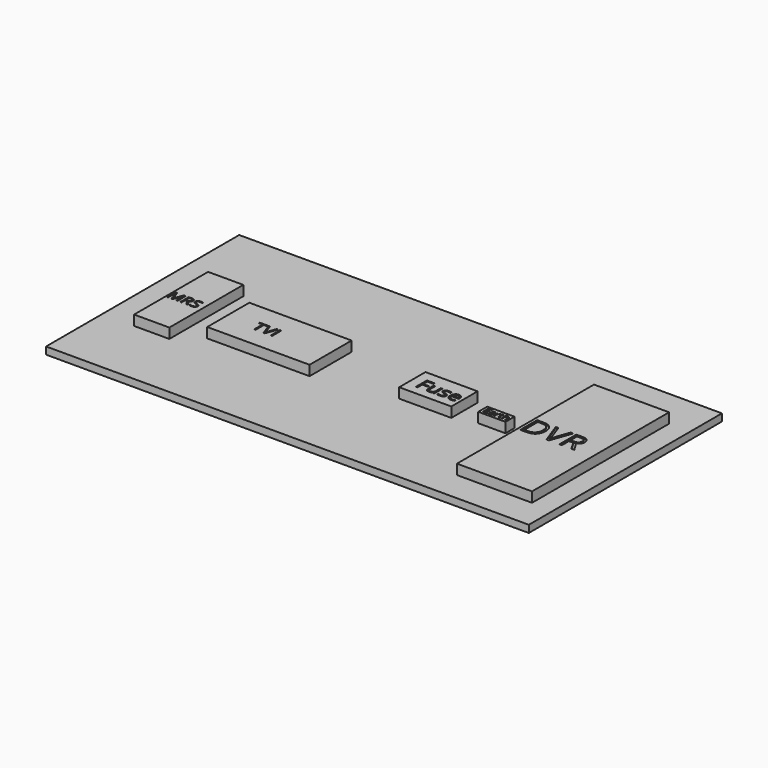
from build123d import *

# Parameters (mm, degrees)
F0_W           = 1200
F0_H           = 600
F1_DEPTH       = 18
F2_W           = 87.5000059605
F2_H           = 229.8333570361
F3_DEPTH       = 25
F2_W_2         = 129.4999942183
F2_H_2         = 81.6666670144
F2_W_3         = 67.6666498184
F2_H_3         = 28.0000008643
F2_W_4         = 186.6666674614
F2_H_4         = 425.8333593607
F2_W_5         = 254.3333470821
F2_H_5         = 130.6666657329
F4_TEXT_SIZE   = 36.9619836025
F4_TEXT_SIZE_2 = 40.6544629691
F4_TEXT_SIZE_3 = 47.9405707059
F4_TEXT_SIZE_4 = 24.5655938569
F4_TEXT_SIZE_5 = 73.4881465788
F5_DEPTH       = 3


# Not quite as in the source:
# - Text() gives the source's letters only with a copy of the font that has no kerning and outlines rounded to 1/6400 em; it was checked with that copy


with BuildPart() as f1:
    # F0 (on Top) → F1 (new body)
    with BuildSketch(Plane.XY):
        Rectangle(F0_W, F0_H)
    extrude(amount=F1_DEPTH)


with BuildPart() as f3:
    # F2 (on face) → F3 (new body)
    with BuildSketch(Plane.XY.offset(18)):
        with Locations((-476.5833467245, -11.0833384097)):
            Rectangle(F2_W, F2_H)
    extrude(amount=F3_DEPTH)


with BuildPart() as f3b:
    # F2 (on face) → F3, piece 2 (new body)
    with BuildSketch(Plane.XY.offset(18)):
        with Locations((137.0833404362, -2.3333337158)):
            Rectangle(F2_W_2, F2_H_2)
    extrude(amount=F3_DEPTH)


with BuildPart() as f3c:
    # F2 (on face) → F3, piece 3 (new body)
    with BuildSketch(Plane.XY.offset(18)):
        with Locations((290.5000150204, -14.0000004321)):
            Rectangle(F2_W_3, F2_H_3)
    extrude(amount=F3_DEPTH)


with BuildPart() as f3d:
    # F2 (on face) → F3, piece 4 (new body)
    with BuildSketch(Plane.XY.offset(18)):
        with Locations((453.8333714008, -11.0833272338)):
            Rectangle(F2_W_4, F2_H_4)
    extrude(amount=F3_DEPTH)


with BuildPart() as f3e:
    # F2 (on face) → F3, piece 5 (new body)
    with BuildSketch(Plane.XY.offset(18)):
        with Locations((-249.6666759253, -12.8333307803)):
            Rectangle(F2_W_5, F2_H_5)
    extrude(amount=F3_DEPTH)


with BuildPart() as f5_tool:
    # F4 (on face) → F5 (new body)
    with BuildSketch(Plane.XY.offset(43)):
        with Locations((-520.3333497047, -28.9940357329)):
            Text('MRS', F4_TEXT_SIZE, font='Open Sans', text_align=(TextAlign.LEFT, TextAlign.BOTTOM))
        with Locations((-309.0552091599, -29.2712133378)):
            Text('TVI', F4_TEXT_SIZE_2, font='Open Sans', text_align=(TextAlign.LEFT, TextAlign.BOTTOM))
        with Locations((91.7636616685, -21.500791423)):
            Text('Fuse', F4_TEXT_SIZE_3, font='Open Sans', text_align=(TextAlign.LEFT, TextAlign.BOTTOM))
        with Locations((260.8784735203, -21.9294135459)):
            Text('Earth', F4_TEXT_SIZE_4, font='Open Sans', text_align=(TextAlign.LEFT, TextAlign.BOTTOM))
        with Locations((360.5000376701, -36.3580513952)):
            Text('DVR', F4_TEXT_SIZE_5, font='Open Sans', text_align=(TextAlign.LEFT, TextAlign.BOTTOM))
    extrude(amount=-F5_DEPTH)


with BuildPart() as f3_1:
    add(f3.part)

    # F5: cut by f5_tool
    add(f5_tool.part, mode=Mode.SUBTRACT)


with BuildPart() as f3b_1:
    add(f3b.part)

    # F5: cut by f5_tool
    add(f5_tool.part, mode=Mode.SUBTRACT)


with BuildPart() as f3c_1:
    add(f3c.part)

    # F5: cut by f5_tool
    add(f5_tool.part, mode=Mode.SUBTRACT)


with BuildPart() as f3d_1:
    add(f3d.part)

    # F5: cut by f5_tool
    add(f5_tool.part, mode=Mode.SUBTRACT)


with BuildPart() as f3e_1:
    add(f3e.part)

    # F5: cut by f5_tool
    add(f5_tool.part, mode=Mode.SUBTRACT)


solid = Compound([f1.part, f3_1.part, f3b_1.part, f3c_1.part, f3d_1.part, f3e_1.part])
